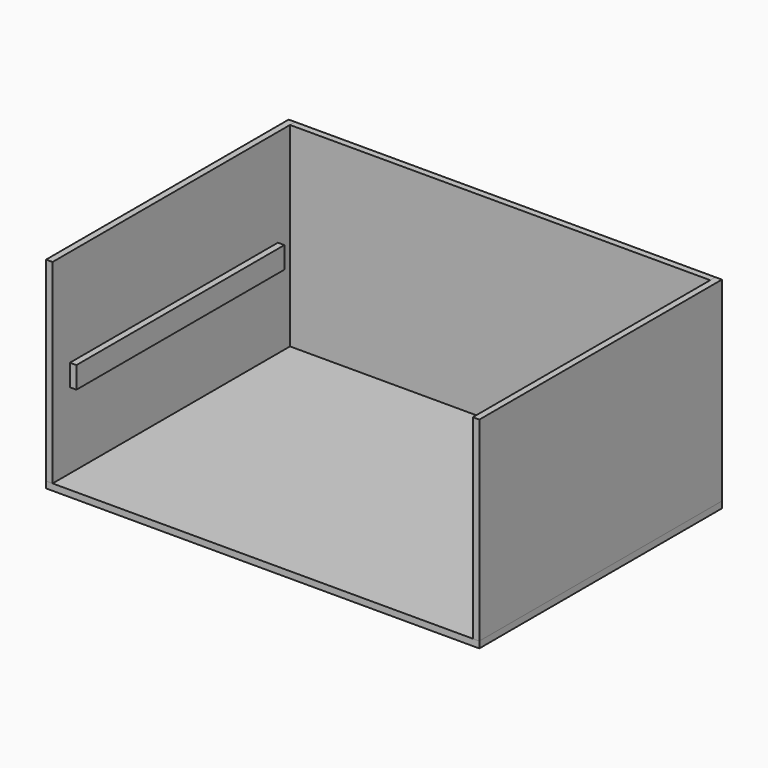
from build123d import *

# Parameters (mm, degrees)
F1_DEPTH = 450
F0_W     = 970
F0_H     = 15
F2_DEPTH = 450
F3_DEPTH = 450
F0_H_2   = 685
F4_DEPTH = 15
F5_DEPTH = 450
F7_DEPTH = 15
F9_DEPTH = 450


# Not quite as in the source:
# - a feature names something its author has since deleted; it is built from what else it names


with BuildPart() as f1:
    # F0 (on Top) → F1 (new body)
    with BuildSketch(Plane.XY):
        Polygon((-500, -350), (-485, -350), (-485, 335), (-485, 350), (-500, 350), align=None)
    extrude(amount=F1_DEPTH)


with BuildPart() as f2:
    # F0 (on Top) → F2 (new body)
    with BuildSketch(Plane.XY):
        with Locations((0, 342.5)):
            Rectangle(F0_W, F0_H)
    extrude(amount=F2_DEPTH)


with BuildPart() as f3:
    # F0 (on Top) → F3 (new body)
    with BuildSketch(Plane.XY):
        Polygon((485, -350), (500, -350), (500, 350), (485, 350), (485, 335), align=None)
    extrude(amount=F3_DEPTH)


with BuildPart() as f4:
    # F0 (on Top) → F4 (new body)
    with BuildSketch(Plane.XY):
        Polygon((-500, -350), (-485, -350), (-485, 335), (-485, 350), (-500, 350), align=None)
        with Locations((0, -7.5)):
            Rectangle(F0_W, F0_H_2)
        with Locations((0, 342.5)):
            Rectangle(F0_W, F0_H)
        Polygon((485, -350), (500, -350), (500, 350), (485, 350), (485, 335), align=None)
    extrude(amount=-F4_DEPTH)


with BuildPart() as f5:
    # F0 (on Top) → F5 (new body)
    with BuildSketch(Plane.XY):
        with Locations((0, 342.5)):
            Rectangle(F0_W, F0_H)
    extrude(amount=F5_DEPTH)


with BuildPart() as f7:
    # F6 (on face) → F7 (new body)
    with BuildSketch(Plane.YZ.offset(-485)):
        Polygon((-300, 175), (0, 175), (300, 175), (300, 225), (-300, 225), align=None)
    extrude(amount=F7_DEPTH)


with BuildPart() as f8_1:
    # F8: instance of F7
    add(f7.part.mirror(Plane.YZ))


with BuildPart() as f9:
    # F0 (on Top) → F9 (new body)
    with BuildSketch(Plane.XY):
        Polygon((-500, -350), (-485, -350), (-485, 335), (-485, 350), (-500, 350), align=None)
    extrude(amount=F9_DEPTH)


solid = Compound([f3.part, f4.part, f5.part, f7.part, f8_1.part, f9.part])
